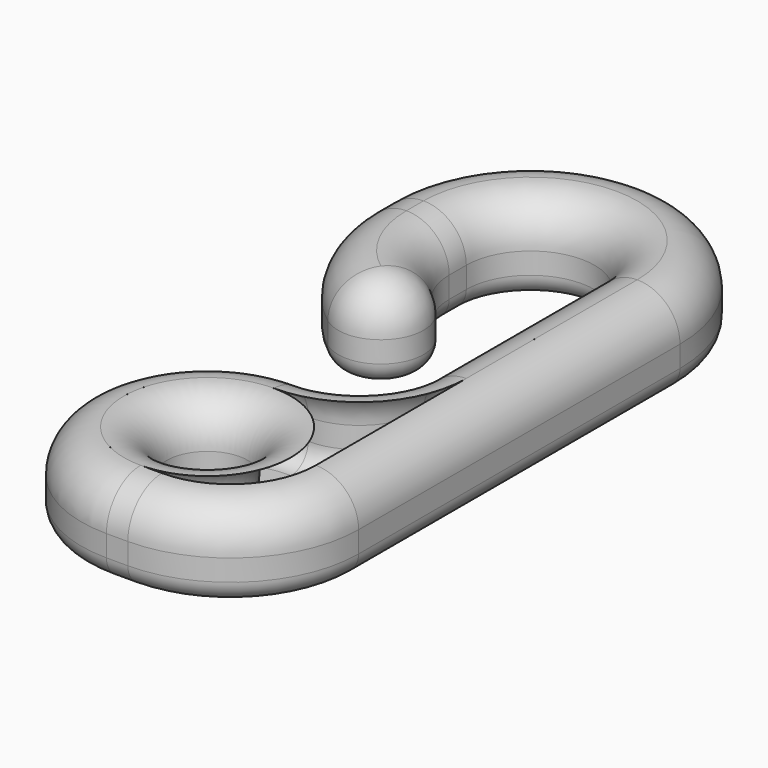
from build123d import *

# Parameters (mm, degrees)
F0_R     = 1.9
F1_DEPTH = 4
F2_R     = 1.99999
F3_R     = 1


# Not quite as in the source:
# - a fillet or chamfer is up to 0.001 mm smaller than in the source, because OpenCascade refuses the exact size


with BuildPart() as f1:
    # F0 (on Top) → F1 (new body)
    with BuildSketch(Plane.XY):
        with BuildLine():
            ThreePointArc((-3, 0), (0, 3), (3, 0))
            Line((3, 0), (3, -10))
            ThreePointArc((3, -10), (2.1213203436, -12.1213203436), (0, -13))
            ThreePointArc((0, -13), (-5.9, -18.9), (0, -24.8))
            Line((0, -24.8), (1, -24.8))
            ThreePointArc((1, -24.8), (5.2426406871, -23.0426406871), (7, -18.8))
            Line((7, -18.8), (7, 0))
            ThreePointArc((7, 0), (0, 7), (-7, 0))
            Line((-7, 0), (-7, -1))
            ThreePointArc((-7, -1), (-6.260990337, -4.1304951685), (-4.2, -6.6))
            ThreePointArc((-4.2, -6.6), (-2.105572809, -6.788854382), (-1, -5))
            ThreePointArc((-1, -5), (-1.211145618, -4.105572809), (-1.8, -3.4))
            ThreePointArc((-1.8, -3.4), (-2.683281573, -2.3416407865), (-3, -1))
            Line((-3, -1), (-3, 0))
        make_face()
        with Locations((0, -18.9)):
            Circle(F0_R, mode=Mode.SUBTRACT)
    extrude(amount=F1_DEPTH)

    # F2 (radius 2 in the source; OpenCascade refuses exactly that, so slightly less here)
    f2_edges = [f1.edges().sort_by_distance(p)[0] for p in [
        (0, 3, 4),
        (-1.9, -18.9, 4),
    ]]
    fillet(f2_edges, radius=F2_R)

    # F3
    f3_edges = [f1.edges().sort_by_distance(p)[0] for p in [
        (7, -9.4, 0),
        (0, 7, 0),
        (-7, -0.5, 0),
    ]]
    fillet(f3_edges, radius=F3_R)


solid = f1.part
